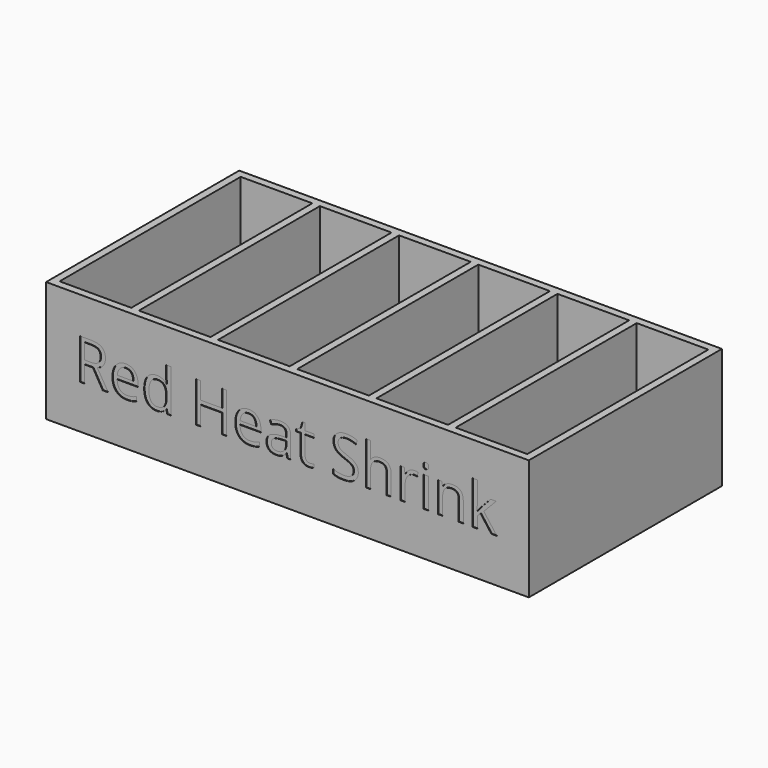
from build123d import *

# Parameters (mm, degrees)
F0_W         = 203.2
F0_H         = 101.6
F0_W_2       = 30.1625
F0_H_2       = 95.25
F1_DEPTH     = 47.625
F2_TEXT_SIZE = 23.8125
F3_DEPTH     = 0.254
F4_W         = 203.2
F4_H         = 101.6
F5_DEPTH     = 3.175


# Not quite as in the source:
# - a feature names something its author has since deleted; it is built from what else it names
# - Text() gives the source's letters only with a copy of the font that has no kerning and outlines rounded to 1/6400 em; it was checked with that copy


with BuildPart() as f1:
    # F0 (on Top) → F1 (new body)
    with BuildSketch(Plane.XY):
        with Locations((101.6, -50.8)):
            Rectangle(F0_W, F0_H)
        with Locations((18.25625, -50.8)):
            Rectangle(F0_W_2, F0_H_2, mode=Mode.SUBTRACT)
        with Locations((51.59375, -50.8)):
            Rectangle(F0_W_2, F0_H_2, mode=Mode.SUBTRACT)
        with Locations((84.93125, -50.8)):
            Rectangle(F0_W_2, F0_H_2, mode=Mode.SUBTRACT)
        Polygon((133.35, -98.425), (103.1875, -98.425), (103.1875, -3.175), (117.0652287364, -3.175), (133.35, -3.175), align=None, mode=Mode.SUBTRACT)
        with Locations((151.60625, -50.8)):
            Rectangle(F0_W_2, F0_H_2, mode=Mode.SUBTRACT)
        with Locations((184.94375, -50.8)):
            Rectangle(F0_W_2, F0_H_2, mode=Mode.SUBTRACT)
    extrude(amount=F1_DEPTH)

    # F2 (on face) → F3 (cut)
    with BuildSketch(Plane.XZ.offset(101.6)):
        with Locations((11.8696630859, 15.24)):
            Text('Red Heat Shrink', F2_TEXT_SIZE, font='Open Sans', text_align=(TextAlign.LEFT, TextAlign.BOTTOM))
    extrude(amount=-F3_DEPTH, mode=Mode.SUBTRACT)

    # F4 (on face) → F5 (join)
    with BuildSketch(Plane(origin=(0, 0, 0), x_dir=(1, 0, 0), z_dir=(0, 0, -1))):
        with Locations((101.6, 50.8)):
            Rectangle(F4_W, F4_H)
    extrude(amount=F5_DEPTH)


solid = f1.part
